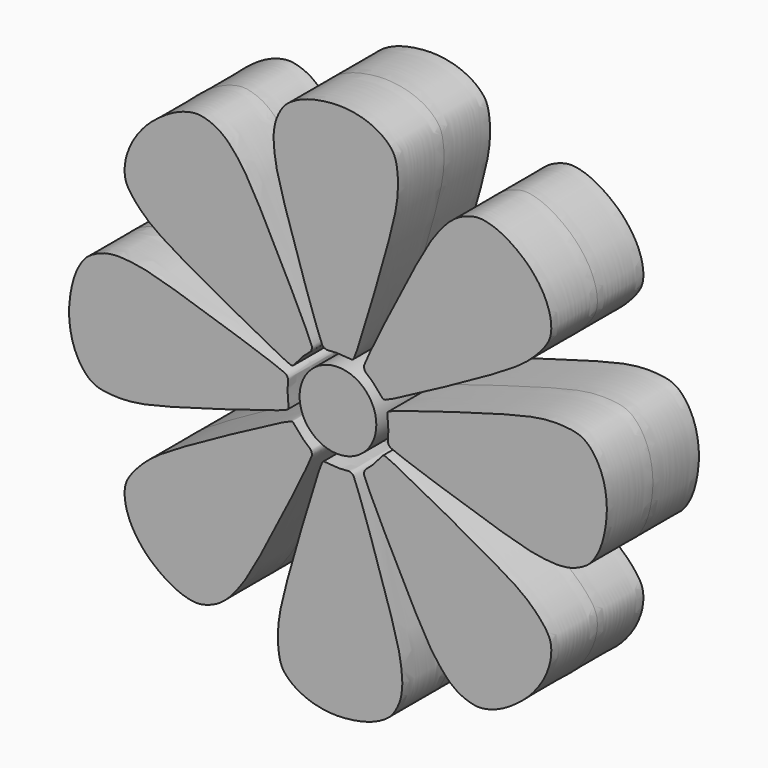
from build123d import *

# Parameters (mm, degrees)
F2_DEPTH = 4.5
F1_R     = 3


# Not quite as in the source:
# - the dataset's text gives a spline's control points without its knots; the knots are read off the source's solid


with BuildPart() as f2:
    # F1 (on Front) → F2 (new body, symmetric)
    with BuildSketch(Plane.XZ):
        with BuildLine():
            add(Edge.make_bspline(
                [(-2.0934587639, 3.4483161563), (-2.0770267358, 3.4856295044), (-2.0042061538, 3.662746157), (-2.1617166196, 4.2472504057), (-6.6666093027, 13.3276848085), (-7.8416898095, 14.8564509472), (-8.6042605194, 15.7724248858), (-9.4534955289, 16.4298537758), (-10.3360809541, 16.7503582254), (-11.0489432081, 16.8904860016), (-11.9504170665, 16.7096665623), (-12.7871647203, 16.3856510787), (-13.735690248, 15.8253847803), (-14.9007679603, 14.9084599984), (-15.7551482495, 13.8473452819), (-16.2754409774, 12.9527263274), (-16.6296276121, 11.9137353584), (-16.7053696977, 11.0446941799), (-16.6100740143, 10.276247164), (-15.9839066339, 9.3497777102), (-15.0167230638, 8.3552803712), (-13.5645820026, 7.2225347631), (-8.6243829296, 4.4811544856), (-3.9867574945, 1.9982562985), (-3.5509117037, 1.9059555674), (-3.437197505, 2.0253329781), (-3.1628367519, 2.3450261924), (-2.7997534438, 2.7900760457), (-2.5293237062, 3.0294303059), (-2.2969999445, 3.2154678163), (-2.1220998785, 3.387927922), (-2.1036259175, 3.4252288941), (-2.0934587639, 3.4483161563)],
                knots=[0, 0, 0, 0, 0.0132047521, 0.0367190386, 0.1380011002, 0.1859973619, 0.2184440513, 0.2515025506, 0.2821887284, 0.3091984365, 0.3393500048, 0.3695710418, 0.4029937495, 0.4421129365, 0.4793775898, 0.5118939754, 0.5451490945, 0.5747911718, 0.6022617235, 0.6355751344, 0.672459156, 0.7146396005, 0.7934842211, 0.8659400752, 0.8828172471, 0.8942458301, 0.9149849552, 0.9396434145, 0.9588430489, 0.9765347292, 0.9918296913, 1, 1, 1, 1], degree=3))
        make_face()
    extrude(amount=F2_DEPTH, both=True)


with BuildPart() as f2b:
    # F1 (on Front) → F2, piece 2 (new body, symmetric)
    with BuildSketch(Plane.XZ):
        with BuildLine():
            add(Edge.make_bspline(
                [(-0.9580288497, 3.9186266259), (-0.9960325697, 3.9333919488), (-1.1727648831, 4.0071404076), (-1.4746950826, 4.531824044), (-4.7100916601, 14.138100951), (-4.9601851688, 16.0500092494), (-5.0686576321, 17.2369195529), (-4.9330302244, 18.3022918132), (-4.535578955, 19.1530048221), (-4.1305945218, 19.7561598567), (-3.3652975919, 20.2657394833), (-2.544514106, 20.6282958778), (-1.4776371744, 20.9028366117), (-0.0054390923, 21.0783072316), (1.3490204156, 20.932123916), (2.349514061, 20.6674353029), (3.334639392, 20.1832055143), (4.0027020448, 19.6222583462), (4.4786919167, 19.0115000263), (4.6910375492, 17.9136199921), (4.7103513004, 16.5265021188), (4.4845046096, 14.6987112264), (2.9297049287, 9.2670143774), (1.4060826801, 4.2320438386), (1.1631596388, 3.8585878514), (0.9983389811, 3.862592347), (0.5782793924, 3.8946472377), (0.0068429538, 3.9526063377), (-0.353628768, 3.9306326569), (-0.6494548604, 3.8979033347), (-0.8950755934, 3.8961780222), (-0.9345144267, 3.9094907295), (-0.9580288497, 3.9186266259)],
                knots=[0, 0, 0, 0, 0.0132047521, 0.0367190386, 0.1380011002, 0.1859973619, 0.2184440513, 0.2515025506, 0.2821887284, 0.3091984365, 0.3393500048, 0.3695710418, 0.4029937495, 0.4421129365, 0.4793775898, 0.5118939754, 0.5451490945, 0.5747911718, 0.6022617235, 0.6355751344, 0.672459156, 0.7146396005, 0.7934842211, 0.8659400752, 0.8828172471, 0.8942458301, 0.9149849552, 0.9396434145, 0.9588430489, 0.9765347292, 0.9918296913, 1, 1, 1, 1], degree=3))
        make_face()
    extrude(amount=F2_DEPTH, both=True)


with BuildPart() as f2c:
    # F1 (on Front) → F2, piece 3 (new body, symmetric)
    with BuildSketch(Plane.XZ):
        with BuildLine():
            add(Edge.make_bspline(
                [(2.0934587639, 3.4483161563), (2.0770267358, 3.4856295044), (2.0042061538, 3.662746157), (2.1617166196, 4.2472504057), (6.6666093027, 13.3276848085), (7.8416898095, 14.8564509472), (8.6042605194, 15.7724248858), (9.4534955289, 16.4298537758), (10.3360809541, 16.7503582254), (11.0489432081, 16.8904860016), (11.9504170665, 16.7096665623), (12.7871647203, 16.3856510787), (13.735690248, 15.8253847803), (14.9007679603, 14.9084599984), (15.7551482495, 13.8473452819), (16.2754409774, 12.9527263274), (16.6296276121, 11.9137353584), (16.7053696977, 11.0446941799), (16.6100740143, 10.276247164), (15.9839066339, 9.3497777102), (15.0167230638, 8.3552803712), (13.5645820026, 7.2225347631), (8.6243829296, 4.4811544856), (3.9867574945, 1.9982562985), (3.5509117037, 1.9059555674), (3.437197505, 2.0253329781), (3.1628367519, 2.3450261924), (2.7997534438, 2.7900760457), (2.5293237062, 3.0294303059), (2.2969999445, 3.2154678163), (2.1220998785, 3.387927922), (2.1036259175, 3.4252288941), (2.0934587639, 3.4483161563)],
                knots=[0, 0, 0, 0, 0.0132047521, 0.0367190386, 0.1380011002, 0.1859973619, 0.2184440513, 0.2515025506, 0.2821887284, 0.3091984365, 0.3393500048, 0.3695710418, 0.4029937495, 0.4421129365, 0.4793775898, 0.5118939754, 0.5451490945, 0.5747911718, 0.6022617235, 0.6355751344, 0.672459156, 0.7146396005, 0.7934842211, 0.8659400752, 0.8828172471, 0.8942458301, 0.9149849552, 0.9396434145, 0.9588430489, 0.9765347292, 0.9918296913, 1, 1, 1, 1], degree=3))
        make_face()
    extrude(amount=F2_DEPTH, both=True)


with BuildPart() as f2d:
    # F1 (on Front) → F2, piece 4 (new body, symmetric)
    with BuildSketch(Plane.XZ):
        with BuildLine():
            add(Edge.make_bspline(
                [(3.9186266259, -0.9580288497), (3.9333919488, -0.9960325697), (4.0071404076, -1.1727648831), (4.531824044, -1.4746950826), (14.138100951, -4.7100916601), (16.0500092494, -4.9601851688), (17.2369195529, -5.0686576321), (18.3022918132, -4.9330302244), (19.1530048221, -4.535578955), (19.7561598567, -4.1305945218), (20.2657394833, -3.3652975919), (20.6282958778, -2.544514106), (20.9028366117, -1.4776371744), (21.0783072316, -0.0054390923), (20.932123916, 1.3490204156), (20.6674353029, 2.349514061), (20.1832055143, 3.334639392), (19.6222583462, 4.0027020448), (19.0115000263, 4.4786919167), (17.9136199921, 4.6910375492), (16.5265021188, 4.7103513004), (14.6987112264, 4.4845046096), (9.2670143774, 2.9297049287), (4.2320438386, 1.4060826801), (3.8585878514, 1.1631596388), (3.862592347, 0.9983389811), (3.8946472377, 0.5782793924), (3.9526063377, 0.0068429538), (3.9306326569, -0.353628768), (3.8979033347, -0.6494548604), (3.8961780222, -0.8950755934), (3.9094907295, -0.9345144267), (3.9186266259, -0.9580288497)],
                knots=[0, 0, 0, 0, 0.0132047521, 0.0367190386, 0.1380011002, 0.1859973619, 0.2184440513, 0.2515025506, 0.2821887284, 0.3091984365, 0.3393500048, 0.3695710418, 0.4029937495, 0.4421129365, 0.4793775898, 0.5118939754, 0.5451490945, 0.5747911718, 0.6022617235, 0.6355751344, 0.672459156, 0.7146396005, 0.7934842211, 0.8659400752, 0.8828172471, 0.8942458301, 0.9149849552, 0.9396434145, 0.9588430489, 0.9765347292, 0.9918296913, 1, 1, 1, 1], degree=3))
        make_face()
    extrude(amount=F2_DEPTH, both=True)


with BuildPart() as f2e:
    # F1 (on Front) → F2, piece 5 (new body, symmetric)
    with BuildSketch(Plane.XZ):
        with BuildLine():
            add(Edge.make_bspline(
                [(2.0934587639, -3.4483161563), (2.0770267358, -3.4856295044), (2.0042061538, -3.662746157), (2.1617166196, -4.2472504057), (6.6666093027, -13.3276848085), (7.8416898095, -14.8564509472), (8.6042605194, -15.7724248858), (9.4534955289, -16.4298537758), (10.3360809541, -16.7503582254), (11.0489432081, -16.8904860016), (11.9504170665, -16.7096665623), (12.7871647203, -16.3856510787), (13.735690248, -15.8253847803), (14.9007679603, -14.9084599984), (15.7551482495, -13.8473452819), (16.2754409774, -12.9527263274), (16.6296276121, -11.9137353584), (16.7053696977, -11.0446941799), (16.6100740143, -10.276247164), (15.9839066339, -9.3497777102), (15.0167230638, -8.3552803712), (13.5645820026, -7.2225347631), (8.6243829296, -4.4811544856), (3.9867574945, -1.9982562985), (3.5509117037, -1.9059555674), (3.437197505, -2.0253329781), (3.1628367519, -2.3450261924), (2.7997534438, -2.7900760457), (2.5293237062, -3.0294303059), (2.2969999445, -3.2154678163), (2.1220998785, -3.387927922), (2.1036259175, -3.4252288941), (2.0934587639, -3.4483161563)],
                knots=[0, 0, 0, 0, 0.0132047521, 0.0367190386, 0.1380011002, 0.1859973619, 0.2184440513, 0.2515025506, 0.2821887284, 0.3091984365, 0.3393500048, 0.3695710418, 0.4029937495, 0.4421129365, 0.4793775898, 0.5118939754, 0.5451490945, 0.5747911718, 0.6022617235, 0.6355751344, 0.672459156, 0.7146396005, 0.7934842211, 0.8659400752, 0.8828172471, 0.8942458301, 0.9149849552, 0.9396434145, 0.9588430489, 0.9765347292, 0.9918296913, 1, 1, 1, 1], degree=3))
        make_face()
    extrude(amount=F2_DEPTH, both=True)


with BuildPart() as f2f:
    # F1 (on Front) → F2, piece 6 (new body, symmetric)
    with BuildSketch(Plane.XZ):
        with BuildLine():
            add(Edge.make_bspline(
                [(0.9580288497, -3.9186266259), (0.9960325697, -3.9333919488), (1.1727648831, -4.0071404076), (1.4746950826, -4.531824044), (4.7100916601, -14.138100951), (4.9601851688, -16.0500092494), (5.0686576321, -17.2369195529), (4.9330302244, -18.3022918132), (4.535578955, -19.1530048221), (4.1305945218, -19.7561598567), (3.3652975919, -20.2657394833), (2.544514106, -20.6282958778), (1.4776371744, -20.9028366117), (0.0054390923, -21.0783072316), (-1.3490204156, -20.932123916), (-2.349514061, -20.6674353029), (-3.334639392, -20.1832055143), (-4.0027020448, -19.6222583462), (-4.4786919167, -19.0115000263), (-4.6910375492, -17.9136199921), (-4.7103513004, -16.5265021188), (-4.4845046096, -14.6987112264), (-2.9297049287, -9.2670143774), (-1.4060826801, -4.2320438386), (-1.1631596388, -3.8585878514), (-0.9983389811, -3.862592347), (-0.5782793924, -3.8946472377), (-0.0068429538, -3.9526063377), (0.353628768, -3.9306326569), (0.6494548604, -3.8979033347), (0.8950755934, -3.8961780222), (0.9345144267, -3.9094907295), (0.9580288497, -3.9186266259)],
                knots=[0, 0, 0, 0, 0.0132047521, 0.0367190386, 0.1380011002, 0.1859973619, 0.2184440513, 0.2515025506, 0.2821887284, 0.3091984365, 0.3393500048, 0.3695710418, 0.4029937495, 0.4421129365, 0.4793775898, 0.5118939754, 0.5451490945, 0.5747911718, 0.6022617235, 0.6355751344, 0.672459156, 0.7146396005, 0.7934842211, 0.8659400752, 0.8828172471, 0.8942458301, 0.9149849552, 0.9396434145, 0.9588430489, 0.9765347292, 0.9918296913, 1, 1, 1, 1], degree=3))
        make_face()
    extrude(amount=F2_DEPTH, both=True)


with BuildPart() as f2g:
    # F1 (on Front) → F2, piece 7 (new body, symmetric)
    with BuildSketch(Plane.XZ):
        with BuildLine():
            add(Edge.make_bspline(
                [(-2.0934587639, -3.4483161563), (-2.0770267358, -3.4856295044), (-2.0042061538, -3.662746157), (-2.1617166196, -4.2472504057), (-6.6666093027, -13.3276848085), (-7.8416898095, -14.8564509472), (-8.6042605194, -15.7724248858), (-9.4534955289, -16.4298537758), (-10.3360809541, -16.7503582254), (-11.0489432081, -16.8904860016), (-11.9504170665, -16.7096665623), (-12.7871647203, -16.3856510787), (-13.735690248, -15.8253847803), (-14.9007679603, -14.9084599984), (-15.7551482495, -13.8473452819), (-16.2754409774, -12.9527263274), (-16.6296276121, -11.9137353584), (-16.7053696977, -11.0446941799), (-16.6100740143, -10.276247164), (-15.9839066339, -9.3497777102), (-15.0167230638, -8.3552803712), (-13.5645820026, -7.2225347631), (-8.6243829296, -4.4811544856), (-3.9867574945, -1.9982562985), (-3.5509117037, -1.9059555674), (-3.437197505, -2.0253329781), (-3.1628367519, -2.3450261924), (-2.7997534438, -2.7900760457), (-2.5293237062, -3.0294303059), (-2.2969999445, -3.2154678163), (-2.1220998785, -3.387927922), (-2.1036259175, -3.4252288941), (-2.0934587639, -3.4483161563)],
                knots=[0, 0, 0, 0, 0.0132047521, 0.0367190386, 0.1380011002, 0.1859973619, 0.2184440513, 0.2515025506, 0.2821887284, 0.3091984365, 0.3393500048, 0.3695710418, 0.4029937495, 0.4421129365, 0.4793775898, 0.5118939754, 0.5451490945, 0.5747911718, 0.6022617235, 0.6355751344, 0.672459156, 0.7146396005, 0.7934842211, 0.8659400752, 0.8828172471, 0.8942458301, 0.9149849552, 0.9396434145, 0.9588430489, 0.9765347292, 0.9918296913, 1, 1, 1, 1], degree=3))
        make_face()
    extrude(amount=F2_DEPTH, both=True)


with BuildPart() as f2h:
    # F1 (on Front) → F2, piece 8 (new body, symmetric)
    with BuildSketch(Plane.XZ):
        with BuildLine():
            add(Edge.make_bspline(
                [(-3.9186266259, 0.9580288497), (-3.9333919488, 0.9960325697), (-4.0071404076, 1.1727648831), (-4.531824044, 1.4746950826), (-14.138100951, 4.7100916601), (-16.0500092494, 4.9601851688), (-17.2369195529, 5.0686576321), (-18.3022918132, 4.9330302244), (-19.1530048221, 4.535578955), (-19.7561598567, 4.1305945218), (-20.2657394833, 3.3652975919), (-20.6282958778, 2.544514106), (-20.9028366117, 1.4776371744), (-21.0783072316, 0.0054390923), (-20.932123916, -1.3490204156), (-20.6674353029, -2.349514061), (-20.1832055143, -3.334639392), (-19.6222583462, -4.0027020448), (-19.0115000263, -4.4786919167), (-17.9136199921, -4.6910375492), (-16.5265021188, -4.7103513004), (-14.6987112264, -4.4845046096), (-9.2670143774, -2.9297049287), (-4.2320438386, -1.4060826801), (-3.8585878514, -1.1631596388), (-3.862592347, -0.9983389811), (-3.8946472377, -0.5782793924), (-3.9526063377, -0.0068429538), (-3.9306326569, 0.353628768), (-3.8979033347, 0.6494548604), (-3.8961780222, 0.8950755934), (-3.9094907295, 0.9345144267), (-3.9186266259, 0.9580288497)],
                knots=[0, 0, 0, 0, 0.0132047521, 0.0367190386, 0.1380011002, 0.1859973619, 0.2184440513, 0.2515025506, 0.2821887284, 0.3091984365, 0.3393500048, 0.3695710418, 0.4029937495, 0.4421129365, 0.4793775898, 0.5118939754, 0.5451490945, 0.5747911718, 0.6022617235, 0.6355751344, 0.672459156, 0.7146396005, 0.7934842211, 0.8659400752, 0.8828172471, 0.8942458301, 0.9149849552, 0.9396434145, 0.9588430489, 0.9765347292, 0.9918296913, 1, 1, 1, 1], degree=3))
        make_face()
    extrude(amount=F2_DEPTH, both=True)


with BuildPart() as f2i:
    # F1 (on Front) → F2, piece 9 (new body, symmetric)
    with BuildSketch(Plane.XZ):
        Circle(F1_R)
    extrude(amount=F2_DEPTH, both=True)


solid = Compound([f2.part, f2b.part, f2c.part, f2d.part, f2e.part, f2f.part, f2g.part, f2h.part, f2i.part])
